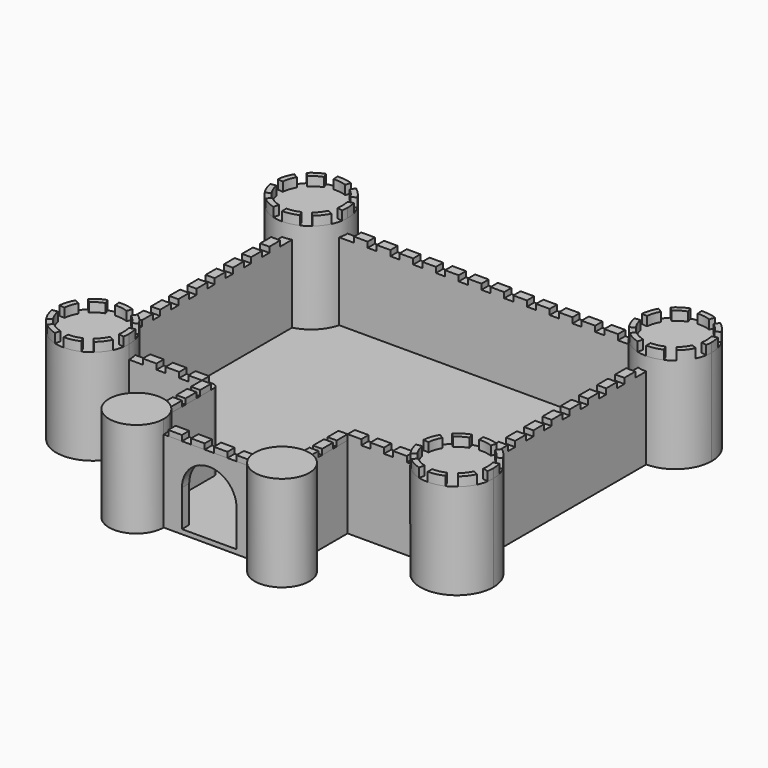
from build123d import *

# Parameters (mm, degrees)
F1_DEPTH  = 6.35
F2_DEPTH  = 133.35
F4_DEPTH  = 107.95
F5_W      = 19.05
F5_H      = 12.7
F6_DEPTH  = 7.62
F7_W      = 12.7
F7_H      = 19.05
F8_DEPTH  = 7.62
F9_W      = 19.05
F9_H      = 12.7
F10_DEPTH = 7.62
F11_W     = 12.7
F11_H     = 19.05
F12_DEPTH = 7.62
F14_DEPTH = 12.7
F16_DEPTH = 12.7
F18_DEPTH = 12.7
F20_DEPTH = 12.7
F21_DEPTH = 114.3
F22_DEPTH = 133.35
F24_DEPTH = 12.7
F25_W     = 12.7
F25_H     = 19.05
F28_DEPTH = 7.62
F26_W     = 19.05
F26_H     = 12.7
F27_W     = 12.7
F27_H     = 19.05
F29_R     = 7.62


# Not quite as in the source:
# - a feature names something its author has since deleted; it is built from what else it names


with BuildPart() as f1:
    # F0 (on Top) → F1 (new body)
    with BuildSketch(Plane.XY):
        with BuildLine():
            Line((326.0391152322, 291.6201265194), (-80.3608847678, 291.6201265194))
            ThreePointArc((-80.3608847678, 291.6201265194), (-95.2398602835, 255.6991020351), (-131.1608847678, 240.8201265194))
            Line((-131.1608847678, 240.8201265194), (-131.1608847678, -38.5798734806))
            ThreePointArc((-131.1608847678, -38.5798734806), (-95.2398602835, -53.4588489964), (-80.3608847678, -89.3798734806))
            Line((-80.3608847678, -89.3798734806), (21.2391152322, -89.3798734806))
            Line((21.2391152322, -89.3798734806), (33.9391152322, -89.3798734806))
            Line((33.9391152322, -89.3798734806), (211.7391152322, -89.3798734806))
            Line((211.7391152322, -89.3798734806), (224.4391152322, -89.3798734806))
            Line((224.4391152322, -89.3798734806), (326.0391152322, -89.3798734806))
            ThreePointArc((326.0391152322, -89.3798734806), (340.918090748, -53.4588489964), (376.8391152322, -38.5798734806))
            Line((376.8391152322, -38.5798734806), (376.8391152322, 240.8201265194))
            ThreePointArc((376.8391152322, 240.8201265194), (340.918090748, 255.6991020351), (326.0391152322, 291.6201265194))
        make_face()
        with BuildLine():
            Line((211.7391152322, -89.3798734806), (33.9391152322, -89.3798734806))
            Line((33.9391152322, -89.3798734806), (33.9391152322, -167.7588489964))
            ThreePointArc((33.9391152322, -167.7588489964), (48.1798835954, -176.7391051174), (57.1601397165, -190.9798734806))
            Line((57.1601397165, -190.9798734806), (188.518090748, -190.9798734806))
            ThreePointArc((188.518090748, -190.9798734806), (197.498346869, -176.7391051174), (211.7391152322, -167.7588489964))
            Line((211.7391152322, -167.7588489964), (211.7391152322, -89.3798734806))
        make_face()
    extrude(amount=F1_DEPTH)

    # F0 (on Top) → F2 (join)
    with BuildSketch(Plane.XY):
        with BuildLine():
            Line((-131.1608847678, 240.8201265194), (-131.1608847678, 291.6201265194))
            Line((-131.1608847678, 291.6201265194), (-80.3608847678, 291.6201265194))
            ThreePointArc((-80.3608847678, 291.6201265194), (-167.081909252, 327.5411510036), (-131.1608847678, 240.8201265194))
        make_face()
        with BuildLine():
            Line((-80.3608847678, 291.6201265194), (-131.1608847678, 291.6201265194))
            Line((-131.1608847678, 291.6201265194), (-131.1608847678, 240.8201265194))
            ThreePointArc((-131.1608847678, 240.8201265194), (-95.2398602835, 255.6991020351), (-80.3608847678, 291.6201265194))
        make_face()
        with BuildLine():
            Line((-131.1608847678, -89.3798734806), (-131.1608847678, -38.5798734806))
            ThreePointArc((-131.1608847678, -38.5798734806), (-167.081909252, -125.3008979649), (-80.3608847678, -89.3798734806))
            Line((-80.3608847678, -89.3798734806), (-131.1608847678, -89.3798734806))
        make_face()
        with BuildLine():
            ThreePointArc((-80.3608847678, -89.3798734806), (-95.2398602835, -53.4588489964), (-131.1608847678, -38.5798734806))
            Line((-131.1608847678, -38.5798734806), (-131.1608847678, -89.3798734806))
            Line((-131.1608847678, -89.3798734806), (-80.3608847678, -89.3798734806))
        make_face()
        with BuildLine():
            Line((376.8391152322, 291.6201265194), (326.0391152322, 291.6201265194))
            ThreePointArc((326.0391152322, 291.6201265194), (340.918090748, 255.6991020351), (376.8391152322, 240.8201265194))
            Line((376.8391152322, 240.8201265194), (376.8391152322, 291.6201265194))
        make_face()
        with BuildLine():
            ThreePointArc((427.6391152322, 291.6201265194), (376.8391152322, 342.4201265194), (326.0391152322, 291.6201265194))
            Line((326.0391152322, 291.6201265194), (376.8391152322, 291.6201265194))
            Line((376.8391152322, 291.6201265194), (376.8391152322, 240.8201265194))
            ThreePointArc((376.8391152322, 240.8201265194), (412.7601397165, 255.6991020351), (427.6391152322, 291.6201265194))
        make_face()
        with BuildLine():
            ThreePointArc((427.6391152322, -89.3798734806), (412.7601397165, -53.4588489964), (376.8391152322, -38.5798734806))
            Line((376.8391152322, -38.5798734806), (376.8391152322, -89.3798734806))
            Line((376.8391152322, -89.3798734806), (326.0391152322, -89.3798734806))
            ThreePointArc((326.0391152322, -89.3798734806), (376.8391152322, -140.1798734806), (427.6391152322, -89.3798734806))
        make_face()
        with BuildLine():
            Line((376.8391152322, -89.3798734806), (376.8391152322, -38.5798734806))
            ThreePointArc((376.8391152322, -38.5798734806), (340.918090748, -53.4588489964), (326.0391152322, -89.3798734806))
            Line((326.0391152322, -89.3798734806), (376.8391152322, -89.3798734806))
        make_face()
    extrude(amount=F2_DEPTH)

    # F3 (on face) → F4 (join)
    with BuildSketch(Plane.XY.offset(6.35)):
        with BuildLine():
            ThreePointArc((-131.1608847678, -38.5798734806), (-124.7598667096, -38.9847649103), (-118.4608847678, -40.1929849838))
            Line((-118.4608847678, -40.1929849838), (-118.4608847678, 242.4332380225))
            ThreePointArc((-118.4608847678, 242.4332380225), (-124.7598667096, 241.225017949), (-131.1608847678, 240.8201265194))
            Line((-131.1608847678, 240.8201265194), (-131.1608847678, -38.5798734806))
        make_face()
        with BuildLine():
            Line((364.1391152322, 242.4332380225), (364.1391152322, -40.1929849838))
            ThreePointArc((364.1391152322, -40.1929849838), (370.4380971741, -38.9847649103), (376.8391152322, -38.5798734806))
            Line((376.8391152322, -38.5798734806), (376.8391152322, 240.8201265194))
            ThreePointArc((376.8391152322, 240.8201265194), (370.4380971741, 241.225017949), (364.1391152322, 242.4332380225))
        make_face()
        with BuildLine():
            ThreePointArc((-80.3608847678, 291.6201265194), (-80.7657761974, 285.2191084612), (-81.9739962709, 278.9201265194))
            Line((-81.9739962709, 278.9201265194), (327.6522267354, 278.9201265194))
            ThreePointArc((327.6522267354, 278.9201265194), (326.4440066619, 285.2191084612), (326.0391152322, 291.6201265194))
            Line((326.0391152322, 291.6201265194), (-80.3608847678, 291.6201265194))
        make_face()
        with BuildLine():
            ThreePointArc((-81.9739962709, -76.6798734806), (-80.7657761974, -82.9788554225), (-80.3608847678, -89.3798734806))
            Line((-80.3608847678, -89.3798734806), (33.9391152322, -89.3798734806))
            Line((33.9391152322, -89.3798734806), (33.9391152322, -76.6798734806))
            Line((33.9391152322, -76.6798734806), (-81.9739962709, -76.6798734806))
        make_face()
        with BuildLine():
            Line((211.7391152322, -76.6798734806), (211.7391152322, -89.3798734806))
            Line((211.7391152322, -89.3798734806), (326.0391152322, -89.3798734806))
            ThreePointArc((326.0391152322, -89.3798734806), (326.4440066619, -82.9788554225), (327.6522267354, -76.6798734806))
            Line((327.6522267354, -76.6798734806), (211.7391152322, -76.6798734806))
        make_face()
    extrude(amount=F4_DEPTH)

    # F5 (on face) → F6 (join)
    with BuildSketch(Plane.XY.offset(114.3)):
        with Locations((-51.7858847678, -83.0298734806)):
            Rectangle(F5_W, F5_H)
        with Locations((-20.0358847678, -83.0298734806)):
            Rectangle(F5_W, F5_H)
        with Locations((11.7141152322, -83.0298734806)):
            Rectangle(F5_W, F5_H)
        with Locations((233.9641152322, -83.0298734806)):
            Rectangle(F5_W, F5_H)
        with Locations((265.7141152322, -83.0298734806)):
            Rectangle(F5_W, F5_H)
        with Locations((297.4641152322, -83.0298734806)):
            Rectangle(F5_W, F5_H)
    extrude(amount=F6_DEPTH)

    # F7 (on face) → F8 (join)
    with BuildSketch(Plane.XY.offset(114.3)):
        with Locations((-124.8108847678, 212.2451265194)):
            Rectangle(F7_W, F7_H)
        with Locations((-124.8108847678, 180.4951265194)):
            Rectangle(F7_W, F7_H)
        with Locations((-124.8108847678, 148.7451265194)):
            Rectangle(F7_W, F7_H)
        with Locations((-124.8108847678, 116.9951265194)):
            Rectangle(F7_W, F7_H)
        with Locations((-124.8108847678, 85.2451265194)):
            Rectangle(F7_W, F7_H)
        with Locations((-124.8108847678, 53.4951265194)):
            Rectangle(F7_W, F7_H)
        with Locations((-124.8108847678, 21.7451265194)):
            Rectangle(F7_W, F7_H)
        with Locations((-124.8108847678, -10.0048734806)):
            Rectangle(F7_W, F7_H)
    extrude(amount=F8_DEPTH)

    # F9 (on face) → F10 (join)
    with BuildSketch(Plane.XY.offset(114.3)):
        with Locations((-51.7858847678, 285.2701265194)):
            Rectangle(F9_W, F9_H)
        with Locations((-20.0358847678, 285.2701265194)):
            Rectangle(F9_W, F9_H)
        with Locations((11.7141152322, 285.2701265194)):
            Rectangle(F9_W, F9_H)
        with Locations((43.4641152322, 285.2701265194)):
            Rectangle(F9_W, F9_H)
        with Locations((75.2141152322, 285.2701265194)):
            Rectangle(F9_W, F9_H)
        with Locations((106.9641152322, 285.2701265194)):
            Rectangle(F9_W, F9_H)
        with Locations((138.7141152322, 285.2701265194)):
            Rectangle(F9_W, F9_H)
        with Locations((170.4641152322, 285.2701265194)):
            Rectangle(F9_W, F9_H)
        with Locations((202.2141152322, 285.2701265194)):
            Rectangle(F9_W, F9_H)
        with Locations((233.9641152322, 285.2701265194)):
            Rectangle(F9_W, F9_H)
        with Locations((265.7141152322, 285.2701265194)):
            Rectangle(F9_W, F9_H)
        with Locations((297.4641152322, 285.2701265194)):
            Rectangle(F9_W, F9_H)
    extrude(amount=F10_DEPTH)

    # F11 (on face) → F12 (join)
    with BuildSketch(Plane.XY.offset(114.3)):
        with Locations((370.4891152322, -10.0048734806)):
            Rectangle(F11_W, F11_H)
        with Locations((370.4891152322, 21.7451265194)):
            Rectangle(F11_W, F11_H)
        with Locations((370.4891152322, 53.4951265194)):
            Rectangle(F11_W, F11_H)
        with Locations((370.4891152322, 85.2451265194)):
            Rectangle(F11_W, F11_H)
        with Locations((370.4891152322, 116.9951265194)):
            Rectangle(F11_W, F11_H)
        with Locations((370.4891152322, 148.7451265194)):
            Rectangle(F11_W, F11_H)
        with Locations((370.4891152322, 180.4951265194)):
            Rectangle(F11_W, F11_H)
        with Locations((370.4891152322, 212.2451265194)):
            Rectangle(F11_W, F11_H)
    extrude(amount=F12_DEPTH)

    # F13 (on face) → F14 (join)
    with BuildSketch(Plane.XY.offset(133.35)):
        with BuildLine():
            ThreePointArc((-161.3553964996, 322.4876476585), (-154.118502096, 328.1914295671), (-145.8361686028, 332.2298352644))
            Line((-145.8361686028, 332.2298352644), (-148.4259245737, 339.3962544547))
            ThreePointArc((-148.4259245737, 339.3962544547), (-158.1698463304, 334.6451889284), (-166.6838397464, 327.9348572713))
            Line((-166.6838397464, 327.9348572713), (-161.3553964996, 322.4876476585))
        make_face()
        with BuildLine():
            ThreePointArc((-134.4252633467, 334.6765573107), (-125.2153238017, 334.3888382699), (-116.276131946, 332.1535267398))
            Line((-116.276131946, 332.1535267398), (-113.6494108598, 339.3064797199))
            ThreePointArc((-113.6494108598, 339.3064797199), (-124.1661071606, 341.9362579905), (-135.0013301548, 342.2747509798))
            Line((-135.0013301548, 342.2747509798), (-134.4252633467, 334.6765573107))
        make_face()
        with BuildLine():
            ThreePointArc((-105.9652829075, 326.6871202157), (-99.1733954219, 320.6255212822), (-93.8032684781, 313.2747081398))
            Line((-93.8032684781, 313.2747081398), (-87.2107479564, 317.0961048963))
            ThreePointArc((-87.2107479564, 317.0961048963), (-93.5285443609, 325.744120358), (-101.5190002263, 332.875413221))
            Line((-101.5190002263, 332.875413221), (-105.9652829075, 326.6871202157))
        make_face()
        with BuildLine():
            ThreePointArc((-89.3687512377, 302.4796833705), (-88.3292567002, 297.09406816), (-87.9808847678, 291.6201265194))
            ThreePointArc((-87.9808847678, 291.6201265194), (-88.1430372849, 287.8815174275), (-88.6282769837, 284.1709873017))
            Line((-88.6282769837, 284.1709873017), (-81.1225226688, 282.8564333221))
            ThreePointArc((-81.1225226688, 282.8564333221), (-80.551652435, 287.2217628819), (-80.3608847678, 291.6201265194))
            ThreePointArc((-80.3608847678, 291.6201265194), (-80.7707341001, 298.0600578613), (-81.99366885, 304.396075756))
            Line((-81.99366885, 304.396075756), (-89.3687512377, 302.4796833705))
        make_face()
        with BuildLine():
            Line((-85.2969637337, 269.7765748992), (-92.1765518888, 273.0531076422))
            ThreePointArc((-92.1765518888, 273.0531076422), (-97.003688858, 265.2042531175), (-103.3862689416, 258.5583190111))
            Line((-103.3862689416, 258.5583190111), (-98.4848661488, 252.7238823921))
            ThreePointArc((-98.4848661488, 252.7238823921), (-90.9759484034, 260.5426283995), (-85.2969637337, 269.7765748992))
        make_face()
        with BuildLine():
            Line((-110.0944680408, 245.3940939588), (-113.2544305499, 252.3279988429))
            ThreePointArc((-113.2544305499, 252.3279988429), (-121.9990528841, 249.4232873423), (-131.1608847678, 248.4401265194))
            Line((-131.1608847678, 248.4401265194), (-131.1608847678, 240.8201265194))
            ThreePointArc((-131.1608847678, 240.8201265194), (-120.3822590222, 241.9767863111), (-110.0944680408, 245.3940939588))
        make_face()
        with BuildLine():
            Line((-144.7646740892, 242.675495393), (-142.724105691, 250.0171900619))
            ThreePointArc((-142.724105691, 250.0171900619), (-151.2880381572, 253.4179001911), (-158.935424598, 258.5582551685))
            Line((-158.935424598, 258.5582551685), (-163.8368139798, 252.7238072831))
            ThreePointArc((-163.8368139798, 252.7238072831), (-154.8398887554, 246.676330839), (-144.7646740892, 242.675495393))
        make_face()
        with BuildLine():
            Line((-173.0594799305, 262.8947418676), (-166.7746906561, 267.2035495653))
            ThreePointArc((-166.7746906561, 267.2035495653), (-171.1444561615, 275.3159424366), (-173.6934583063, 284.170791771))
            Line((-173.6934583063, 284.170791771), (-181.1992065777, 282.8562032859))
            ThreePointArc((-181.1992065777, 282.8562032859), (-178.2003805251, 272.4387334808), (-173.0594799305, 262.8947418676))
        make_face()
        with BuildLine():
            ThreePointArc((-174.1349064843, 295.8327097539), (-172.2626194545, 304.8549217858), (-168.5186503821, 313.2744505288))
            Line((-168.5186503821, 313.2744505288), (-175.1111972552, 317.0958018246))
            ThreePointArc((-175.1111972552, 317.0958018246), (-179.5158667521, 307.1904738916), (-181.7185573754, 296.5761067953))
            Line((-181.7185573754, 296.5761067953), (-174.1349064843, 295.8327097539))
        make_face()
    extrude(amount=F14_DEPTH)

    # F15 (on face) → F16 (join)
    with BuildSketch(Plane.XY.offset(133.35)):
        with BuildLine():
            ThreePointArc((402.0347170925, 326.6871202157), (408.8266045781, 320.6255212822), (414.1967315219, 313.2747081398))
            Line((414.1967315219, 313.2747081398), (420.7892520436, 317.0961048963))
            ThreePointArc((420.7892520436, 317.0961048963), (414.4714556391, 325.744120358), (406.4809997737, 332.875413221))
            Line((406.4809997737, 332.875413221), (402.0347170925, 326.6871202157))
        make_face()
        with BuildLine():
            ThreePointArc((373.5747366533, 334.6765573107), (382.7846761983, 334.3888382699), (391.723868054, 332.1535267398))
            Line((391.723868054, 332.1535267398), (394.3505891402, 339.3064797199))
            ThreePointArc((394.3505891402, 339.3064797199), (383.8338928394, 341.9362579905), (372.9986698452, 342.2747509798))
            Line((372.9986698452, 342.2747509798), (373.5747366533, 334.6765573107))
        make_face()
        with BuildLine():
            ThreePointArc((346.6446035004, 322.4876476585), (353.881497904, 328.1914295671), (362.1638313972, 332.2298352644))
            Line((362.1638313972, 332.2298352644), (359.5740754263, 339.3962544547))
            ThreePointArc((359.5740754263, 339.3962544547), (349.8301536696, 334.6451889284), (341.3161602536, 327.9348572713))
            Line((341.3161602536, 327.9348572713), (346.6446035004, 322.4876476585))
        make_face()
        with BuildLine():
            ThreePointArc((333.8650935157, 295.8327097539), (335.7373805455, 304.8549217858), (339.4813496179, 313.2744505288))
            Line((339.4813496179, 313.2744505288), (332.8888027448, 317.0958018246))
            ThreePointArc((332.8888027448, 317.0958018246), (328.4841332479, 307.1904738916), (326.2814426246, 296.5761067953))
            Line((326.2814426246, 296.5761067953), (333.8650935157, 295.8327097539))
        make_face()
        with BuildLine():
            Line((334.9405200695, 262.8947418676), (341.2253093439, 267.2035495653))
            ThreePointArc((341.2253093439, 267.2035495653), (336.8555438385, 275.3159424366), (334.3065416937, 284.170791771))
            Line((334.3065416937, 284.170791771), (326.8007934223, 282.8562032859))
            ThreePointArc((326.8007934223, 282.8562032859), (329.7996194749, 272.4387334808), (334.9405200695, 262.8947418676))
        make_face()
        with BuildLine():
            Line((363.2353259108, 242.675495393), (365.275894309, 250.0171900619))
            ThreePointArc((365.275894309, 250.0171900619), (356.7119618428, 253.4179001911), (349.064575402, 258.5582551685))
            Line((349.064575402, 258.5582551685), (344.1631860202, 252.7238072831))
            ThreePointArc((344.1631860202, 252.7238072831), (353.1601112446, 246.676330839), (363.2353259108, 242.675495393))
        make_face()
        with BuildLine():
            Line((397.9055319592, 245.3940939588), (394.7455694501, 252.3279988429))
            ThreePointArc((394.7455694501, 252.3279988429), (386.0009471159, 249.4232873423), (376.8391152322, 248.4401265194))
            Line((376.8391152322, 248.4401265194), (376.8391152322, 240.8201265194))
            ThreePointArc((376.8391152322, 240.8201265194), (387.6177409778, 241.9767863111), (397.9055319592, 245.3940939588))
        make_face()
        with BuildLine():
            Line((422.7030362663, 269.7765748992), (415.8234481112, 273.0531076422))
            ThreePointArc((415.8234481112, 273.0531076422), (410.996311142, 265.2042531175), (404.6137310584, 258.5583190111))
            Line((404.6137310584, 258.5583190111), (409.5151338512, 252.7238823921))
            ThreePointArc((409.5151338512, 252.7238823921), (417.0240515966, 260.5426283995), (422.7030362663, 269.7765748992))
        make_face()
        with BuildLine():
            ThreePointArc((418.6312487623, 302.4796833705), (419.6707432998, 297.09406816), (420.0191152322, 291.6201265194))
            ThreePointArc((420.0191152322, 291.6201265194), (419.8569627151, 287.8815174275), (419.3717230163, 284.1709873017))
            Line((419.3717230163, 284.1709873017), (426.8774773312, 282.8564333221))
            ThreePointArc((426.8774773312, 282.8564333221), (427.448347565, 287.2217628819), (427.6391152322, 291.6201265194))
            ThreePointArc((427.6391152322, 291.6201265194), (427.2292658999, 298.0600578613), (426.00633115, 304.396075756))
            Line((426.00633115, 304.396075756), (418.6312487623, 302.4796833705))
        make_face()
    extrude(amount=F16_DEPTH)

    # F17 (on face) → F18 (join)
    with BuildSketch(Plane.XY.offset(133.35)):
        with BuildLine():
            ThreePointArc((-161.3553964996, -58.5123523415), (-154.118502096, -52.8085704329), (-145.8361686028, -48.7701647356))
            Line((-145.8361686028, -48.7701647356), (-148.4259245737, -41.6037455453))
            ThreePointArc((-148.4259245737, -41.6037455453), (-158.1698463304, -46.3548110716), (-166.6838397464, -53.0651427287))
            Line((-166.6838397464, -53.0651427287), (-161.3553964996, -58.5123523415))
        make_face()
        with BuildLine():
            ThreePointArc((-174.1349064843, -85.1672902461), (-172.2626194545, -76.1450782142), (-168.5186503821, -67.7255494712))
            Line((-168.5186503821, -67.7255494712), (-175.1111972552, -63.9041981754))
            ThreePointArc((-175.1111972552, -63.9041981754), (-179.5158667521, -73.8095261084), (-181.7185573754, -84.4238932047))
            Line((-181.7185573754, -84.4238932047), (-174.1349064843, -85.1672902461))
        make_face()
        with BuildLine():
            Line((-173.0594799305, -118.1052581324), (-166.7746906561, -113.7964504347))
            ThreePointArc((-166.7746906561, -113.7964504347), (-171.1444561615, -105.6840575634), (-173.6934583063, -96.829208229))
            Line((-173.6934583063, -96.829208229), (-181.1992065777, -98.1437967141))
            ThreePointArc((-181.1992065777, -98.1437967141), (-178.2003805251, -108.5612665192), (-173.0594799305, -118.1052581324))
        make_face()
        with BuildLine():
            Line((-144.7646740892, -138.324504607), (-142.724105691, -130.9828099381))
            ThreePointArc((-142.724105691, -130.9828099381), (-151.2880381572, -127.5820998089), (-158.935424598, -122.4417448315))
            Line((-158.935424598, -122.4417448315), (-163.8368139798, -128.2761927169))
            ThreePointArc((-163.8368139798, -128.2761927169), (-154.8398887554, -134.323669161), (-144.7646740892, -138.324504607))
        make_face()
        with BuildLine():
            Line((-110.0944680408, -135.6059060412), (-113.2544305499, -128.6720011571))
            ThreePointArc((-113.2544305499, -128.6720011571), (-121.9990528841, -131.5767126577), (-131.1608847678, -132.5598734806))
            Line((-131.1608847678, -132.5598734806), (-131.1608847678, -140.1798734806))
            ThreePointArc((-131.1608847678, -140.1798734806), (-120.3822590222, -139.0232136889), (-110.0944680408, -135.6059060412))
        make_face()
        with BuildLine():
            Line((-85.2969637337, -111.2234251008), (-92.1765518888, -107.9468923578))
            ThreePointArc((-92.1765518888, -107.9468923578), (-97.003688858, -115.7957468825), (-103.3862689416, -122.4416809889))
            Line((-103.3862689416, -122.4416809889), (-98.4848661488, -128.2761176079))
            ThreePointArc((-98.4848661488, -128.2761176079), (-90.9759484034, -120.4573716005), (-85.2969637337, -111.2234251008))
        make_face()
        with BuildLine():
            ThreePointArc((-89.3687512377, -78.5203166295), (-88.3292567002, -83.90593184), (-87.9808847678, -89.3798734806))
            ThreePointArc((-87.9808847678, -89.3798734806), (-88.1430372849, -93.1184825725), (-88.6282769837, -96.8290126983))
            Line((-88.6282769837, -96.8290126983), (-81.1225226688, -98.1435666779))
            ThreePointArc((-81.1225226688, -98.1435666779), (-80.551652435, -93.7782371181), (-80.3608847678, -89.3798734806))
            ThreePointArc((-80.3608847678, -89.3798734806), (-80.7707341001, -82.9399421387), (-81.99366885, -76.603924244))
            Line((-81.99366885, -76.603924244), (-89.3687512377, -78.5203166295))
        make_face()
        with BuildLine():
            ThreePointArc((-105.9652829075, -54.3128797843), (-99.1733954219, -60.3744787178), (-93.8032684781, -67.7252918602))
            Line((-93.8032684781, -67.7252918602), (-87.2107479564, -63.9038951037))
            ThreePointArc((-87.2107479564, -63.9038951037), (-93.5285443609, -55.255879642), (-101.5190002263, -48.124586779))
            Line((-101.5190002263, -48.124586779), (-105.9652829075, -54.3128797843))
        make_face()
        with BuildLine():
            ThreePointArc((-134.4252633467, -46.3234426893), (-125.2153238017, -46.6111617301), (-116.276131946, -48.8464732602))
            Line((-116.276131946, -48.8464732602), (-113.6494108598, -41.6935202801))
            ThreePointArc((-113.6494108598, -41.6935202801), (-124.1661071606, -39.0637420095), (-135.0013301548, -38.7252490202))
            Line((-135.0013301548, -38.7252490202), (-134.4252633467, -46.3234426893))
        make_face()
    extrude(amount=F18_DEPTH)

    # F19 (on face) → F20 (join)
    with BuildSketch(Plane.XY.offset(133.35)):
        with BuildLine():
            ThreePointArc((346.6446035004, -58.5123523415), (353.881497904, -52.8085704329), (362.1638313972, -48.7701647356))
            Line((362.1638313972, -48.7701647356), (359.5740754263, -41.6037455453))
            ThreePointArc((359.5740754263, -41.6037455453), (349.8301536696, -46.3548110716), (341.3161602536, -53.0651427287))
            Line((341.3161602536, -53.0651427287), (346.6446035004, -58.5123523415))
        make_face()
        with BuildLine():
            ThreePointArc((333.8650935157, -85.1672902461), (335.7373805455, -76.1450782142), (339.4813496179, -67.7255494712))
            Line((339.4813496179, -67.7255494712), (332.8888027448, -63.9041981754))
            ThreePointArc((332.8888027448, -63.9041981754), (328.4841332479, -73.8095261084), (326.2814426246, -84.4238932047))
            Line((326.2814426246, -84.4238932047), (333.8650935157, -85.1672902461))
        make_face()
        with BuildLine():
            Line((334.9405200695, -118.1052581324), (341.2253093439, -113.7964504347))
            ThreePointArc((341.2253093439, -113.7964504347), (336.8555438385, -105.6840575634), (334.3065416937, -96.829208229))
            Line((334.3065416937, -96.829208229), (326.8007934223, -98.1437967141))
            ThreePointArc((326.8007934223, -98.1437967141), (329.7996194749, -108.5612665192), (334.9405200695, -118.1052581324))
        make_face()
        with BuildLine():
            Line((363.2353259108, -138.324504607), (365.275894309, -130.9828099381))
            ThreePointArc((365.275894309, -130.9828099381), (356.7119618428, -127.5820998089), (349.064575402, -122.4417448315))
            Line((349.064575402, -122.4417448315), (344.1631860202, -128.2761927169))
            ThreePointArc((344.1631860202, -128.2761927169), (353.1601112446, -134.323669161), (363.2353259108, -138.324504607))
        make_face()
        with BuildLine():
            Line((397.9055319592, -135.6059060412), (394.7455694501, -128.6720011571))
            ThreePointArc((394.7455694501, -128.6720011571), (386.0009471159, -131.5767126577), (376.8391152322, -132.5598734806))
            Line((376.8391152322, -132.5598734806), (376.8391152322, -140.1798734806))
            ThreePointArc((376.8391152322, -140.1798734806), (387.6177409778, -139.0232136889), (397.9055319592, -135.6059060412))
        make_face()
        with BuildLine():
            Line((422.7030362663, -111.2234251008), (415.8234481112, -107.9468923578))
            ThreePointArc((415.8234481112, -107.9468923578), (410.996311142, -115.7957468825), (404.6137310584, -122.4416809889))
            Line((404.6137310584, -122.4416809889), (409.5151338512, -128.2761176079))
            ThreePointArc((409.5151338512, -128.2761176079), (417.0240515966, -120.4573716005), (422.7030362663, -111.2234251008))
        make_face()
        with BuildLine():
            ThreePointArc((418.6312487623, -78.5203166295), (419.6707432998, -83.90593184), (420.0191152322, -89.3798734806))
            ThreePointArc((420.0191152322, -89.3798734806), (419.8569627151, -93.1184825725), (419.3717230163, -96.8290126983))
            Line((419.3717230163, -96.8290126983), (426.8774773312, -98.1435666779))
            ThreePointArc((426.8774773312, -98.1435666779), (427.448347565, -93.7782371181), (427.6391152322, -89.3798734806))
            ThreePointArc((427.6391152322, -89.3798734806), (427.2292658999, -82.9399421387), (426.00633115, -76.603924244))
            Line((426.00633115, -76.603924244), (418.6312487623, -78.5203166295))
        make_face()
        with BuildLine():
            ThreePointArc((402.0347170925, -54.3128797843), (408.8266045781, -60.3744787178), (414.1967315219, -67.7252918602))
            Line((414.1967315219, -67.7252918602), (420.7892520436, -63.9038951037))
            ThreePointArc((420.7892520436, -63.9038951037), (414.4714556391, -55.255879642), (406.4809997737, -48.124586779))
            Line((406.4809997737, -48.124586779), (402.0347170925, -54.3128797843))
        make_face()
        with BuildLine():
            ThreePointArc((373.5747366533, -46.3234426893), (382.7846761983, -46.6111617301), (391.723868054, -48.8464732602))
            Line((391.723868054, -48.8464732602), (394.3505891402, -41.6935202801))
            ThreePointArc((394.3505891402, -41.6935202801), (383.8338928394, -39.0637420095), (372.9986698452, -38.7252490202))
            Line((372.9986698452, -38.7252490202), (373.5747366533, -46.3234426893))
        make_face()
    extrude(amount=F20_DEPTH)

    # F0 (on Top) → F21 (join)
    with BuildSketch(Plane.XY):
        with BuildLine():
            Line((33.9391152322, -89.3798734806), (21.2391152322, -89.3798734806))
            Line((21.2391152322, -89.3798734806), (21.2391152322, -165.5798734806))
            ThreePointArc((21.2391152322, -165.5798734806), (27.6819006217, -166.1285683578), (33.9391152322, -167.7588489964))
            Line((33.9391152322, -167.7588489964), (33.9391152322, -89.3798734806))
        make_face()
        with BuildLine():
            ThreePointArc((57.1601397165, -190.9798734806), (58.790420355, -197.2370880912), (59.3391152322, -203.6798734806))
            Line((59.3391152322, -203.6798734806), (186.3391152322, -203.6798734806))
            ThreePointArc((186.3391152322, -203.6798734806), (186.8878101094, -197.2370880912), (188.518090748, -190.9798734806))
            Line((188.518090748, -190.9798734806), (57.1601397165, -190.9798734806))
        make_face()
        with BuildLine():
            Line((224.4391152322, -165.5798734806), (224.4391152322, -89.3798734806))
            Line((224.4391152322, -89.3798734806), (211.7391152322, -89.3798734806))
            Line((211.7391152322, -89.3798734806), (211.7391152322, -167.7588489964))
            ThreePointArc((211.7391152322, -167.7588489964), (217.9963298428, -166.1285683578), (224.4391152322, -165.5798734806))
        make_face()
    extrude(amount=F21_DEPTH)

    # F23 (on face) → F24 (cut)
    with BuildSketch(Plane.XZ.offset(203.6798734806)):
        with BuildLine():
            ThreePointArc((160.9391152322, 57.15), (122.8391152322, 95.25), (84.7391152322, 57.15))
            Line((84.7391152322, 57.15), (84.7391152322, 6.35))
            Line((84.7391152322, 6.35), (160.9391152322, 6.35))
            Line((160.9391152322, 6.35), (160.9391152322, 57.15))
        make_face()
    extrude(amount=-F24_DEPTH, mode=Mode.SUBTRACT)

    # F29
    f29_edges = [f1.edges().sort_by_distance(p)[0] for p in [
        (211.739115, -76.679873, 60.325),
        (33.939115, -76.679873, 60.325),
    ]]
    fillet(f29_edges, radius=F29_R)


with BuildPart() as f22:
    # F0 (on Top) → F22 (new body)
    with BuildSketch(Plane.XY):
        with BuildLine():
            Line((21.2391152322, -203.6798734806), (21.2391152322, -165.5798734806))
            ThreePointArc((21.2391152322, -165.5798734806), (-5.701653131, -230.6206418439), (59.3391152322, -203.6798734806))
            Line((59.3391152322, -203.6798734806), (21.2391152322, -203.6798734806))
        make_face()
        with BuildLine():
            ThreePointArc((57.1601397165, -190.9798734806), (48.1798835954, -176.7391051174), (33.9391152322, -167.7588489964))
            Line((33.9391152322, -167.7588489964), (33.9391152322, -190.9798734806))
            Line((33.9391152322, -190.9798734806), (57.1601397165, -190.9798734806))
        make_face()
        with BuildLine():
            ThreePointArc((33.9391152322, -167.7588489964), (27.6819006217, -166.1285683578), (21.2391152322, -165.5798734806))
            Line((21.2391152322, -165.5798734806), (21.2391152322, -203.6798734806))
            Line((21.2391152322, -203.6798734806), (59.3391152322, -203.6798734806))
            ThreePointArc((59.3391152322, -203.6798734806), (58.790420355, -197.2370880912), (57.1601397165, -190.9798734806))
            Line((57.1601397165, -190.9798734806), (33.9391152322, -190.9798734806))
            Line((33.9391152322, -190.9798734806), (33.9391152322, -167.7588489964))
        make_face()
    extrude(amount=F22_DEPTH)


with BuildPart() as f22b:
    # F0 (on Top) → F22, piece 2 (new body)
    with BuildSketch(Plane.XY):
        with BuildLine():
            ThreePointArc((262.5391152322, -203.6798734806), (251.3798835954, -176.7391051174), (224.4391152322, -165.5798734806))
            Line((224.4391152322, -165.5798734806), (224.4391152322, -203.6798734806))
            Line((224.4391152322, -203.6798734806), (186.3391152322, -203.6798734806))
            ThreePointArc((186.3391152322, -203.6798734806), (224.4391152322, -241.7798734806), (262.5391152322, -203.6798734806))
        make_face()
        with BuildLine():
            Line((224.4391152322, -203.6798734806), (224.4391152322, -165.5798734806))
            ThreePointArc((224.4391152322, -165.5798734806), (217.9963298428, -166.1285683578), (211.7391152322, -167.7588489964))
            Line((211.7391152322, -167.7588489964), (211.7391152322, -190.9798734806))
            Line((211.7391152322, -190.9798734806), (188.518090748, -190.9798734806))
            ThreePointArc((188.518090748, -190.9798734806), (186.8878101094, -197.2370880912), (186.3391152322, -203.6798734806))
            Line((186.3391152322, -203.6798734806), (224.4391152322, -203.6798734806))
        make_face()
        with BuildLine():
            Line((211.7391152322, -190.9798734806), (211.7391152322, -167.7588489964))
            ThreePointArc((211.7391152322, -167.7588489964), (197.498346869, -176.7391051174), (188.518090748, -190.9798734806))
            Line((188.518090748, -190.9798734806), (211.7391152322, -190.9798734806))
        make_face()
    extrude(amount=F22_DEPTH)


with BuildPart() as f28:
    # F25 (on face) → F28 (new body)
    with BuildSketch(Plane.XY.offset(114.3)):
        with Locations((27.5891152322, -98.9048734806)):
            Rectangle(F25_W, F25_H)
    extrude(amount=F28_DEPTH)


with BuildPart() as f28b:
    # F25 (on face) → F28, piece 2 (new body)
    with BuildSketch(Plane.XY.offset(114.3)):
        with Locations((27.5891152322, -124.3048734806)):
            Rectangle(F25_W, F25_H)
    extrude(amount=F28_DEPTH)


with BuildPart() as f28c:
    # F25 (on face) → F28, piece 3 (new body)
    with BuildSketch(Plane.XY.offset(114.3)):
        with Locations((27.5891152322, -149.7048734806)):
            Rectangle(F25_W, F25_H)
    extrude(amount=F28_DEPTH)


with BuildPart() as f28d:
    # F26 (on face) → F28, piece 4 (new body)
    with BuildSketch(Plane.XY.offset(114.3)):
        with Locations((75.2141152322, -197.3298734806)):
            Rectangle(F26_W, F26_H)
    extrude(amount=F28_DEPTH)


with BuildPart() as f28e:
    # F26 (on face) → F28, piece 5 (new body)
    with BuildSketch(Plane.XY.offset(114.3)):
        with Locations((106.9641152322, -197.3298734806)):
            Rectangle(F26_W, F26_H)
    extrude(amount=F28_DEPTH)


with BuildPart() as f28f:
    # F26 (on face) → F28, piece 6 (new body)
    with BuildSketch(Plane.XY.offset(114.3)):
        with Locations((138.7141152322, -197.3298734806)):
            Rectangle(F26_W, F26_H)
    extrude(amount=F28_DEPTH)


with BuildPart() as f28g:
    # F26 (on face) → F28, piece 7 (new body)
    with BuildSketch(Plane.XY.offset(114.3)):
        with Locations((170.4641152322, -197.3298734806)):
            Rectangle(F26_W, F26_H)
    extrude(amount=F28_DEPTH)


with BuildPart() as f28h:
    # F27 (on face) → F28, piece 8 (new body)
    with BuildSketch(Plane.XY.offset(114.3)):
        with Locations((218.0891152322, -149.7048734806)):
            Rectangle(F27_W, F27_H)
    extrude(amount=F28_DEPTH)


with BuildPart() as f28i:
    # F27 (on face) → F28, piece 9 (new body)
    with BuildSketch(Plane.XY.offset(114.3)):
        with Locations((218.0891152322, -124.3048734806)):
            Rectangle(F27_W, F27_H)
    extrude(amount=F28_DEPTH)


with BuildPart() as f28j:
    # F27 (on face) → F28, piece 10 (new body)
    with BuildSketch(Plane.XY.offset(114.3)):
        with Locations((218.0891152322, -98.9048734806)):
            Rectangle(F27_W, F27_H)
    extrude(amount=F28_DEPTH)


solid = Compound([f1.part, f22.part, f22b.part, f28.part, f28b.part, f28c.part, f28d.part, f28e.part, f28f.part, f28g.part, f28h.part, f28i.part, f28j.part])
